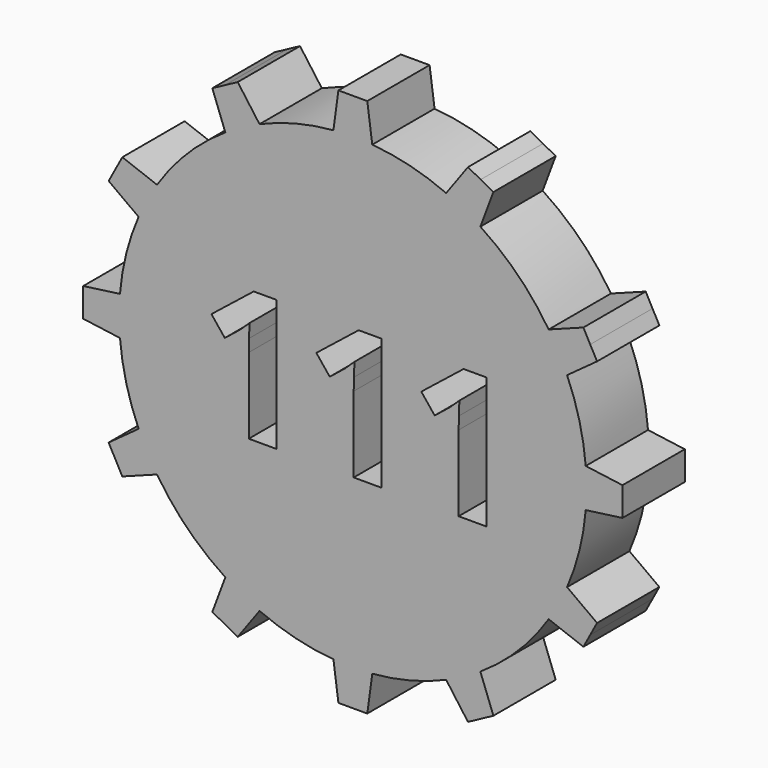
from build123d import *

# Parameters (mm, degrees)
F1_DEPTH     = 3.175
F2_TEXT_SIZE = 7.4939071459
F3_DEPTH     = 25.4


# Not quite as in the source:
# - Text() gives the source's letters only with a copy of the font that has no kerning and outlines rounded to 1/6400 em; it was checked with that copy


with BuildPart() as f1:
    # F0 (on Front) → F1 (new body)
    with BuildSketch(Plane.XZ):
        with BuildLine():
            Line((-9.525, 0), (0, 0))
            Line((0, 0), (-8.3862150663, 4.5163062189))
            ThreePointArc((-8.3862150663, 4.5163062189), (-8.5667814141, 4.163637977), (-8.7325249862, 3.8037655508))
            ThreePointArc((-8.7325249862, 3.8037655508), (-9.2359169416, 2.3288330226), (-9.4920527683, 0.7915549533))
            ThreePointArc((-9.4920527683, 0.7915549533), (-9.5167596276, 0.3961201725), (-9.525, 0))
        make_face()
        with BuildLine():
            Line((-8.3862150663, 4.5163062189), (0, 0))
            Line((0, 0), (-4.5163062189, 8.3862150663))
            ThreePointArc((-4.5163062189, 8.3862150663), (-4.861160068, 8.1911383698), (-5.197602837, 7.9818888584))
            ThreePointArc((-5.197602837, 7.9818888584), (-6.7351920908, 6.7351920908), (-7.9818888584, 5.197602837))
            ThreePointArc((-7.9818888584, 5.197602837), (-8.1911383698, 4.861160068), (-8.3862150663, 4.5163062189))
        make_face()
        with BuildLine():
            Line((0, 9.525), (0, 0))
            Line((0, 0), (4.5163062189, 8.3862150663))
            ThreePointArc((4.5163062189, 8.3862150663), (4.163637977, 8.5667814141), (3.8037655508, 8.7325249862))
            ThreePointArc((3.8037655508, 8.7325249862), (2.3288330226, 9.2359169416), (0.7915549533, 9.4920527683))
            ThreePointArc((0.7915549533, 9.4920527683), (0.3961201725, 9.5167596276), (0, 9.525))
        make_face()
        with BuildLine():
            Line((-4.5163062189, 8.3862150663), (0, 0))
            Line((0, 0), (0, 9.525))
            ThreePointArc((0, 9.525), (-0.3961201725, 9.5167596276), (-0.7915549533, 9.4920527683))
            ThreePointArc((-0.7915549533, 9.4920527683), (-2.3288330226, 9.2359169416), (-3.8037655508, 8.7325249862))
            ThreePointArc((-3.8037655508, 8.7325249862), (-4.163637977, 8.5667814141), (-4.5163062189, 8.3862150663))
        make_face()
        with BuildLine():
            Line((4.5163062189, 8.3862150663), (0, 0))
            Line((0, 0), (8.3862150663, 4.5163062189))
            ThreePointArc((8.3862150663, 4.5163062189), (8.1911383698, 4.861160068), (7.9818888584, 5.197602837))
            ThreePointArc((7.9818888584, 5.197602837), (6.7351920908, 6.7351920908), (5.197602837, 7.9818888584))
            ThreePointArc((5.197602837, 7.9818888584), (4.861160068, 8.1911383698), (4.5163062189, 8.3862150663))
        make_face()
        with BuildLine():
            Line((0, 0), (9.525, 0))
            ThreePointArc((9.525, 0), (9.5167596276, 0.3961201725), (9.4920527683, 0.7915549533))
            ThreePointArc((9.4920527683, 0.7915549533), (9.2359169416, 2.3288330226), (8.7325249862, 3.8037655508))
            ThreePointArc((8.7325249862, 3.8037655508), (8.5667814141, 4.163637977), (8.3862150663, 4.5163062189))
            Line((8.3862150663, 4.5163062189), (0, 0))
        make_face()
        with BuildLine():
            ThreePointArc((9.4920527683, -0.7915549533), (9.5167596276, -0.3961201725), (9.525, 0))
            Line((9.525, 0), (0, 0))
            Line((0, 0), (8.3862150663, -4.5163062189))
            ThreePointArc((8.3862150663, -4.5163062189), (8.5667814141, -4.163637977), (8.7325249862, -3.8037655508))
            ThreePointArc((8.7325249862, -3.8037655508), (9.2359169416, -2.3288330226), (9.4920527683, -0.7915549533))
        make_face()
        with BuildLine():
            Line((8.3862150663, -4.5163062189), (0, 0))
            Line((0, 0), (4.5163062189, -8.3862150663))
            ThreePointArc((4.5163062189, -8.3862150663), (4.861160068, -8.1911383698), (5.197602837, -7.9818888584))
            ThreePointArc((5.197602837, -7.9818888584), (6.7351920908, -6.7351920908), (7.9818888584, -5.197602837))
            ThreePointArc((7.9818888584, -5.197602837), (8.1911383698, -4.861160068), (8.3862150663, -4.5163062189))
        make_face()
        with BuildLine():
            Line((4.5163062189, -8.3862150663), (0, 0))
            Line((0, 0), (0, -9.525))
            ThreePointArc((0, -9.525), (0.3961201725, -9.5167596276), (0.7915549533, -9.4920527683))
            ThreePointArc((0.7915549533, -9.4920527683), (2.3288330226, -9.2359169416), (3.8037655508, -8.7325249862))
            ThreePointArc((3.8037655508, -8.7325249862), (4.163637977, -8.5667814141), (4.5163062189, -8.3862150663))
        make_face()
        with BuildLine():
            Line((0, -9.525), (0, 0))
            Line((0, 0), (-4.5163062189, -8.3862150663))
            ThreePointArc((-4.5163062189, -8.3862150663), (-4.163637977, -8.5667814141), (-3.8037655508, -8.7325249862))
            ThreePointArc((-3.8037655508, -8.7325249862), (-2.3288330226, -9.2359169416), (-0.7915549533, -9.4920527683))
            ThreePointArc((-0.7915549533, -9.4920527683), (-0.3961201725, -9.5167596276), (0, -9.525))
        make_face()
        with BuildLine():
            Line((-4.5163062189, -8.3862150663), (0, 0))
            Line((0, 0), (-8.3862150663, -4.5163062189))
            ThreePointArc((-8.3862150663, -4.5163062189), (-8.1911383698, -4.861160068), (-7.9818888584, -5.197602837))
            ThreePointArc((-7.9818888584, -5.197602837), (-6.7351920908, -6.7351920908), (-5.197602837, -7.9818888584))
            ThreePointArc((-5.197602837, -7.9818888584), (-4.861160068, -8.1911383698), (-4.5163062189, -8.3862150663))
        make_face()
        with BuildLine():
            Line((-8.3862150663, -4.5163062189), (0, 0))
            Line((0, 0), (-9.525, 0))
            ThreePointArc((-9.525, 0), (-9.5167596276, -0.3961201725), (-9.4920527683, -0.7915549533))
            ThreePointArc((-9.4920527683, -0.7915549533), (-9.2359169416, -2.3288330226), (-8.7325249862, -3.8037655508))
            ThreePointArc((-8.7325249862, -3.8037655508), (-8.5667814141, -4.163637977), (-8.3862150663, -4.5163062189))
        make_face()
        with BuildLine():
            Line((-10.9892907151, 0), (-9.525, 0))
            ThreePointArc((-9.525, 0), (-9.5167596276, 0.3961201725), (-9.4920527683, 0.7915549533))
            Line((-9.4920527683, 0.7915549533), (-10.9892907151, 0.58829693))
            Line((-10.9892907151, 0.58829693), (-10.9892907151, 0))
        make_face()
        with BuildLine():
            ThreePointArc((-9.4920527683, -0.7915549533), (-9.5167596276, -0.3961201725), (-9.525, 0))
            Line((-9.525, 0), (-10.9892907151, 0))
            Line((-10.9892907151, 0), (-10.9892907151, -0.58829693))
            Line((-10.9892907151, -0.58829693), (-9.4920527683, -0.7915549533))
        make_face()
        with BuildLine():
            ThreePointArc((-8.7325249862, 3.8037655508), (-8.5667814141, 4.163637977), (-8.3862150663, 4.5163062189))
            Line((-8.3862150663, 4.5163062189), (-9.6754388832, 5.2106038842))
            Line((-9.6754388832, 5.2106038842), (-9.9543815691, 4.6926422487))
            Line((-9.9543815691, 4.6926422487), (-8.7325249862, 3.8037655508))
        make_face()
        with BuildLine():
            Line((-9.6754388832, 5.2106038842), (-8.3862150663, 4.5163062189))
            ThreePointArc((-8.3862150663, 4.5163062189), (-8.1911383698, 4.861160068), (-7.9818888584, 5.197602837))
            Line((-7.9818888584, 5.197602837), (-9.3964961972, 5.7285655197))
            Line((-9.3964961972, 5.7285655197), (-9.6754388832, 5.2106038842))
        make_face()
        with BuildLine():
            ThreePointArc((-5.197602837, 7.9818888584), (-4.861160068, 8.1911383698), (-4.5163062189, 8.3862150663))
            Line((-4.5163062189, 8.3862150663), (-5.2106038842, 9.6754388832))
            Line((-5.2106038842, 9.6754388832), (-5.7285655197, 9.3964961972))
            Line((-5.7285655197, 9.3964961972), (-5.197602837, 7.9818888584))
        make_face()
        with BuildLine():
            Line((-5.2106038842, 9.6754388832), (-4.5163062189, 8.3862150663))
            ThreePointArc((-4.5163062189, 8.3862150663), (-4.163637977, 8.5667814141), (-3.8037655508, 8.7325249862))
            Line((-3.8037655508, 8.7325249862), (-4.6926422487, 9.9543815691))
            Line((-4.6926422487, 9.9543815691), (-5.2106038842, 9.6754388832))
        make_face()
        with BuildLine():
            ThreePointArc((-0.7915549533, 9.4920527683), (-0.3961201725, 9.5167596276), (0, 9.525))
            Line((0, 9.525), (0, 10.9892907151))
            Line((0, 10.9892907151), (-0.58829693, 10.9892907151))
            Line((-0.58829693, 10.9892907151), (-0.7915549533, 9.4920527683))
        make_face()
        with BuildLine():
            Line((0, 10.9892907151), (0, 9.525))
            ThreePointArc((0, 9.525), (0.3961201725, 9.5167596276), (0.7915549533, 9.4920527683))
            Line((0.7915549533, 9.4920527683), (0.58829693, 10.9892907151))
            Line((0.58829693, 10.9892907151), (0, 10.9892907151))
        make_face()
        with BuildLine():
            ThreePointArc((3.8037655508, 8.7325249862), (4.163637977, 8.5667814141), (4.5163062189, 8.3862150663))
            Line((4.5163062189, 8.3862150663), (5.2106038842, 9.6754388832))
            Line((5.2106038842, 9.6754388832), (4.6926422487, 9.9543815691))
            Line((4.6926422487, 9.9543815691), (3.8037655508, 8.7325249862))
        make_face()
        with BuildLine():
            Line((5.2106038842, 9.6754388832), (4.5163062189, 8.3862150663))
            ThreePointArc((4.5163062189, 8.3862150663), (4.861160068, 8.1911383698), (5.197602837, 7.9818888584))
            Line((5.197602837, 7.9818888584), (5.7285655197, 9.3964961972))
            Line((5.7285655197, 9.3964961972), (5.2106038842, 9.6754388832))
        make_face()
        with BuildLine():
            ThreePointArc((7.9818888584, 5.197602837), (8.1911383698, 4.861160068), (8.3862150663, 4.5163062189))
            Line((8.3862150663, 4.5163062189), (9.6754388832, 5.2106038842))
            Line((9.6754388832, 5.2106038842), (9.3964961972, 5.7285655197))
            Line((9.3964961972, 5.7285655197), (7.9818888584, 5.197602837))
        make_face()
        with BuildLine():
            ThreePointArc((8.3862150663, 4.5163062189), (8.5667814141, 4.163637977), (8.7325249862, 3.8037655508))
            Line((8.7325249862, 3.8037655508), (9.9543815691, 4.6926422487))
            Line((9.9543815691, 4.6926422487), (9.6754388832, 5.2106038842))
            Line((9.6754388832, 5.2106038842), (8.3862150663, 4.5163062189))
        make_face()
        with BuildLine():
            ThreePointArc((9.4920527683, 0.7915549533), (9.5167596276, 0.3961201725), (9.525, 0))
            Line((9.525, 0), (10.9892907151, 0))
            Line((10.9892907151, 0), (10.9892907151, 0.58829693))
            Line((10.9892907151, 0.58829693), (9.4920527683, 0.7915549533))
        make_face()
        with BuildLine():
            Line((10.9892907151, 0), (9.525, 0))
            ThreePointArc((9.525, 0), (9.5167596276, -0.3961201725), (9.4920527683, -0.7915549533))
            Line((9.4920527683, -0.7915549533), (10.9892907151, -0.58829693))
            Line((10.9892907151, -0.58829693), (10.9892907151, 0))
        make_face()
        with BuildLine():
            Line((9.9543815691, -4.6926422487), (8.7325249862, -3.8037655508))
            ThreePointArc((8.7325249862, -3.8037655508), (8.5667814141, -4.163637977), (8.3862150663, -4.5163062189))
            Line((8.3862150663, -4.5163062189), (9.6754388832, -5.2106038842))
            Line((9.6754388832, -5.2106038842), (9.9543815691, -4.6926422487))
        make_face()
        with BuildLine():
            Line((9.6754388832, -5.2106038842), (8.3862150663, -4.5163062189))
            ThreePointArc((8.3862150663, -4.5163062189), (8.1911383698, -4.861160068), (7.9818888584, -5.197602837))
            Line((7.9818888584, -5.197602837), (9.3964961972, -5.7285655197))
            Line((9.3964961972, -5.7285655197), (9.6754388832, -5.2106038842))
        make_face()
        with BuildLine():
            ThreePointArc((5.197602837, -7.9818888584), (4.861160068, -8.1911383698), (4.5163062189, -8.3862150663))
            Line((4.5163062189, -8.3862150663), (5.2106038842, -9.6754388832))
            Line((5.2106038842, -9.6754388832), (5.7285655197, -9.3964961972))
            Line((5.7285655197, -9.3964961972), (5.197602837, -7.9818888584))
        make_face()
        with BuildLine():
            Line((5.2106038842, -9.6754388832), (4.5163062189, -8.3862150663))
            ThreePointArc((4.5163062189, -8.3862150663), (4.163637977, -8.5667814141), (3.8037655508, -8.7325249862))
            Line((3.8037655508, -8.7325249862), (4.6926422487, -9.9543815691))
            Line((4.6926422487, -9.9543815691), (5.2106038842, -9.6754388832))
        make_face()
        with BuildLine():
            ThreePointArc((0.7915549533, -9.4920527683), (0.3961201725, -9.5167596276), (0, -9.525))
            Line((0, -9.525), (0, -10.9892907151))
            Line((0, -10.9892907151), (0.58829693, -10.9892907151))
            Line((0.58829693, -10.9892907151), (0.7915549533, -9.4920527683))
        make_face()
        with BuildLine():
            Line((0, -10.9892907151), (0, -9.525))
            ThreePointArc((0, -9.525), (-0.3961201725, -9.5167596276), (-0.7915549533, -9.4920527683))
            Line((-0.7915549533, -9.4920527683), (-0.58829693, -10.9892907151))
            Line((-0.58829693, -10.9892907151), (0, -10.9892907151))
        make_face()
        with BuildLine():
            ThreePointArc((-3.8037655508, -8.7325249862), (-4.163637977, -8.5667814141), (-4.5163062189, -8.3862150663))
            Line((-4.5163062189, -8.3862150663), (-5.2106038842, -9.6754388832))
            Line((-5.2106038842, -9.6754388832), (-4.6926422487, -9.9543815691))
            Line((-4.6926422487, -9.9543815691), (-3.8037655508, -8.7325249862))
        make_face()
        with BuildLine():
            Line((-5.2106038842, -9.6754388832), (-4.5163062189, -8.3862150663))
            ThreePointArc((-4.5163062189, -8.3862150663), (-4.861160068, -8.1911383698), (-5.197602837, -7.9818888584))
            Line((-5.197602837, -7.9818888584), (-5.7285655197, -9.3964961972))
            Line((-5.7285655197, -9.3964961972), (-5.2106038842, -9.6754388832))
        make_face()
        with BuildLine():
            ThreePointArc((-7.9818888584, -5.197602837), (-8.1911383698, -4.861160068), (-8.3862150663, -4.5163062189))
            Line((-8.3862150663, -4.5163062189), (-9.6754388832, -5.2106038842))
            Line((-9.6754388832, -5.2106038842), (-9.3964961972, -5.7285655197))
            Line((-9.3964961972, -5.7285655197), (-7.9818888584, -5.197602837))
        make_face()
        with BuildLine():
            Line((-9.6754388832, -5.2106038842), (-8.3862150663, -4.5163062189))
            ThreePointArc((-8.3862150663, -4.5163062189), (-8.5667814141, -4.163637977), (-8.7325249862, -3.8037655508))
            Line((-8.7325249862, -3.8037655508), (-9.9543815691, -4.6926422487))
            Line((-9.9543815691, -4.6926422487), (-9.6754388832, -5.2106038842))
        make_face()
    extrude(amount=F1_DEPTH)

    # F2 (on face) → F3 (cut)
    with BuildSketch(Plane.XZ.offset(3.175)):
        with Locations((-6.2070228159, -2.6978065725)):
            Text('111', F2_TEXT_SIZE, font='Open Sans', font_style=FontStyle.BOLD, text_align=(TextAlign.LEFT, TextAlign.BOTTOM))
    extrude(amount=-F3_DEPTH, mode=Mode.SUBTRACT)


solid = f1.part
